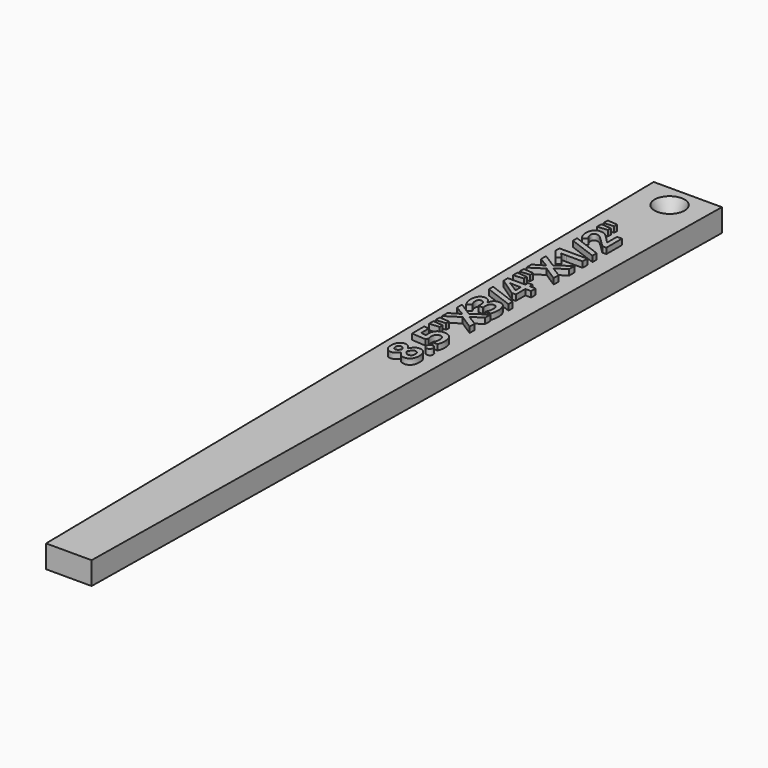
from build123d import *

# Parameters (mm, degrees)
F0_R         = 1.651
F1_DEPTH     = 6.35
F0_TEXT_SIZE = 10.8787272539
F2_DEPTH     = 1.5875
F3_SIZE2     = 2.54
F3_SIZE      = 5.842
F4_DEPTH     = 6.35


# Not quite as in the source:
# - Text() gives the source's letters only with a copy of the font that has no kerning and outlines rounded to 1/6400 em; it was checked with that copy


with BuildPart() as f1:
    # F0 (on Top) → F1 (new body)
    with BuildSketch(Plane.XY):
        Polygon((-35.2317076462, 101.3994294825), (-44.7541336775, 101.3994294825), (-54.2765597088, 101.3994294825), (-51.1044226587, -114.5005705175), (-44.7541336775, -114.5005705175), (-38.4038446963, -114.5005705175), align=None)
        Polygon((-48.8141954362, 16.2280014208), (-48.8141954362, 17.7102280092), (-46.0095235661, 17.490953663), (-46.0095235661, 16.4455759659), align=None, mode=Mode.SUBTRACT)
        Polygon((-48.8141954362, 18.4683393147), (-48.8141954362, 19.950565903), (-46.0095235661, 19.732991358), (-46.0095235661, 18.6876136609), align=None, mode=Mode.SUBTRACT)
        with BuildLine():
            add(Edge.make_bspline(
                [(-48.3994439597, 1.312246475), (-48.9144837031, 2.0023657352), (-48.9144837031, 3.1123358753)],
                knots=[0, 0, 0, 1, 1, 1], degree=2))
            add(Edge.make_bspline(
                [(-48.9144837031, 3.1123358753), (-48.9144837031, 4.22910522), (-48.4070930648, 4.911575375)],
                knots=[0, 0, 0, 1, 1, 1], degree=2))
            add(Edge.make_bspline(
                [(-48.4070930648, 4.911575375), (-47.8997024264, 5.5940455301), (-47.0396030529, 5.5940455301)],
                knots=[0, 0, 0, 1, 1, 1], degree=2))
            add(Edge.make_bspline(
                [(-47.0396030529, 5.5940455301), (-46.4446726562, 5.5940455301), (-45.9797770462, 5.2642841102)],
                knots=[0, 0, 0, 1, 1, 1], degree=2))
            add(Edge.make_bspline(
                [(-45.9797770462, 5.2642841102), (-45.5148814362, 4.9345226903), (-45.1494241926, 4.2019084018)],
                knots=[0, 0, 0, 1, 1, 1], degree=2))
            add(Edge.make_bspline(
                [(-45.1494241926, 4.2019084018), (-44.6819788809, 5.0722065821), (-44.1745882425, 5.4521121355)],
                knots=[0, 0, 0, 1, 1, 1], degree=2))
            add(Edge.make_bspline(
                [(-44.1745882425, 5.4521121355), (-43.6671976042, 5.8320176888), (-43.0603685996, 5.8320176888)],
                knots=[0, 0, 0, 1, 1, 1], degree=2))
            add(Edge.make_bspline(
                [(-43.0603685996, 5.8320176888), (-42.1050803626, 5.8320176888), (-41.5228984744, 5.0832552895)],
                knots=[0, 0, 0, 1, 1, 1], degree=2))
            add(Edge.make_bspline(
                [(-41.5228984744, 5.0832552895), (-40.9407165862, 4.3344928902), (-40.9407165862, 3.1123358753)],
                knots=[0, 0, 0, 1, 1, 1], degree=2))
            add(Edge.make_bspline(
                [(-40.9407165862, 3.1123358753), (-40.9407165862, 1.8374850252), (-41.4829531478, 1.1099701401)],
                knots=[0, 0, 0, 1, 1, 1], degree=2))
            add(Edge.make_bspline(
                [(-41.4829531478, 1.1099701401), (-42.0251897093, 0.382455255), (-43.0178735712, 0.382455255)],
                knots=[0, 0, 0, 1, 1, 1], degree=2))
            add(Edge.make_bspline(
                [(-43.0178735712, 0.382455255), (-43.6824958144, 0.382455255), (-44.1975355578, 0.7360138908)],
                knots=[0, 0, 0, 1, 1, 1], degree=2))
            add(Edge.make_bspline(
                [(-44.1975355578, 0.7360138908), (-44.7125753013, 1.0895725265), (-45.1069291642, 1.8697812468)],
                knots=[0, 0, 0, 1, 1, 1], degree=2))
            add(Edge.make_bspline(
                [(-45.1069291642, 1.8697812468), (-45.525080243, 1.2051590036), (-46.0035742621, 0.9136431092)],
                knots=[0, 0, 0, 1, 1, 1], degree=2))
            add(Edge.make_bspline(
                [(-46.0035742621, 0.9136431092), (-46.4820682812, 0.6221272148), (-47.0498018597, 0.6221272148)],
                knots=[0, 0, 0, 1, 1, 1], degree=2))
            add(Edge.make_bspline(
                [(-47.0498018597, 0.6221272148), (-47.8844042162, 0.6221272148), (-48.3994439597, 1.312246475)],
                knots=[0, 0, 0, 1, 1, 1], degree=2))
        make_face(mode=Mode.SUBTRACT)
        with BuildLine():
            add(Edge.make_bspline(
                [(-45.9347323162, 11.771122849), (-46.0095235661, 12.0957848655), (-46.0095235661, 12.573428984)],
                knots=[0, 0, 0, 1, 1, 1], degree=2))
            add(Edge.make_bspline(
                [(-46.0095235661, 12.573428984), (-46.0095235661, 13.6986973343), (-45.3771975444, 14.3658692792)],
                knots=[0, 0, 0, 1, 1, 1], degree=2))
            add(Edge.make_bspline(
                [(-45.3771975444, 14.3658692792), (-44.7448715228, 15.033041224), (-43.6451001895, 15.033041224)],
                knots=[0, 0, 0, 1, 1, 1], degree=2))
            add(Edge.make_bspline(
                [(-43.6451001895, 15.033041224), (-42.3447523224, 15.033041224), (-41.6427344543, 14.2307350891)],
                knots=[0, 0, 0, 1, 1, 1], degree=2))
            add(Edge.make_bspline(
                [(-41.6427344543, 14.2307350891), (-40.9407165862, 13.4284289541), (-40.9407165862, 11.9360035589)],
                knots=[0, 0, 0, 1, 1, 1], degree=2))
            add(Edge.make_bspline(
                [(-40.9407165862, 11.9360035589), (-40.9407165862, 10.6390552941), (-41.3605674661, 9.8435483637)],
                knots=[0, 0, 0, 1, 1, 1], degree=2))
            Line((-41.3605674661, 9.8435483637), (-42.7799014126, 9.8435483637))
            add(Edge.make_bspline(
                [(-42.7799014126, 9.8435483637), (-42.5572274641, 10.2616994425), (-42.41614397, 10.8200841148)],
                knots=[0, 0, 0, 1, 1, 1], degree=2))
            add(Edge.make_bspline(
                [(-42.41614397, 10.8200841148), (-42.2750604759, 11.3784687872), (-42.2750604759, 11.8765105193)],
                knots=[0, 0, 0, 1, 1, 1], degree=2))
            add(Edge.make_bspline(
                [(-42.2750604759, 11.8765105193), (-42.2750604759, 13.3808345223), (-43.5074162977, 13.3808345223)],
                knots=[0, 0, 0, 1, 1, 1], degree=2))
            add(Edge.make_bspline(
                [(-43.5074162977, 13.3808345223), (-44.6819788809, 13.3808345223), (-44.6819788809, 11.8238166841)],
                knots=[0, 0, 0, 1, 1, 1], degree=2))
            add(Edge.make_bspline(
                [(-44.6819788809, 11.8238166841), (-44.6819788809, 11.5433494971), (-44.6258854435, 11.2033892704)],
                knots=[0, 0, 0, 1, 1, 1], degree=2))
            add(Edge.make_bspline(
                [(-44.6258854435, 11.2033892704), (-44.5697920061, 10.8634290437), (-44.505199563, 10.6509539021)],
                knots=[0, 0, 0, 1, 1, 1], degree=2))
            Line((-44.505199563, 10.6509539021), (-44.8570583976, 9.9965304657))
            Line((-44.8570583976, 9.9965304657), (-48.8141954362, 10.2888962606))
            Line((-48.8141954362, 10.2888962606), (-48.8141954362, 14.5010034693))
            Line((-48.8141954362, 14.5010034693), (-47.422058308, 14.5010034693))
            Line((-47.422058308, 14.5010034693), (-47.422058308, 11.7286278207))
            Line((-47.422058308, 11.7286278207), (-45.8973366913, 11.5858445254))
            Line((-45.8973366913, 11.5858445254), (-45.9347323162, 11.771122849))
        make_face(mode=Mode.SUBTRACT)
        Polygon((-48.8141954362, 45.5342727623), (-48.8141954362, 47.0164993506), (-46.0095235661, 46.7972250044), (-46.0095235661, 45.7518473074), align=None, mode=Mode.SUBTRACT)
        Polygon((-44.9624460679, 25.2896412631), (-41.0478040576, 27.9141342132), (-41.0478040576, 26.0341541596), (-43.9850604162, 24.2272655548), (-41.0478040576, 22.4220767511), (-41.0478040576, 20.6576831746), (-45.052535528, 23.2345816928), (-48.8141954362, 20.8225638845), (-48.8141954362, 22.6396512961), (-46.0197223729, 24.3122556114), (-48.8141954362, 25.9542635063), (-48.8141954362, 27.7271560885), align=None, mode=Mode.SUBTRACT)
        with BuildLine():
            add(Edge.make_bspline(
                [(-48.435989684, 32.7772652559), (-47.9472968582, 33.4758835217), (-47.0769986779, 33.4758835217)],
                knots=[0, 0, 0, 1, 1, 1], degree=2))
            add(Edge.make_bspline(
                [(-47.0769986779, 33.4758835217), (-46.3494837928, 33.4758835217), (-45.8395434527, 33.0347851276)],
                knots=[0, 0, 0, 1, 1, 1], degree=2))
            add(Edge.make_bspline(
                [(-45.8395434527, 33.0347851276), (-45.3296031127, 32.5936867335), (-45.1375255846, 31.7964800019)],
                knots=[0, 0, 0, 1, 1, 1], degree=2))
            Line((-45.1375255846, 31.7964800019), (-45.1069291642, 31.7964800019))
            add(Edge.make_bspline(
                [(-45.1069291642, 31.7964800019), (-44.989642886, 32.7381698298), (-44.5349460828, 33.2209133517)],
                knots=[0, 0, 0, 1, 1, 1], degree=2))
            add(Edge.make_bspline(
                [(-44.5349460828, 33.2209133517), (-44.0802492796, 33.7036568736), (-43.3102393662, 33.7036568736)],
                knots=[0, 0, 0, 1, 1, 1], degree=2))
            add(Edge.make_bspline(
                [(-43.3102393662, 33.7036568736), (-42.1900704193, 33.7036568736), (-41.5653935027, 32.8911519318)],
                knots=[0, 0, 0, 1, 1, 1], degree=2))
            add(Edge.make_bspline(
                [(-41.5653935027, 32.8911519318), (-40.9407165862, 32.0786469901), (-40.9407165862, 30.5709233847)],
                knots=[0, 0, 0, 1, 1, 1], degree=2))
            add(Edge.make_bspline(
                [(-40.9407165862, 30.5709233847), (-40.9407165862, 29.3062713414), (-41.3605674661, 28.3288856897)],
                knots=[0, 0, 0, 1, 1, 1], degree=2))
            Line((-41.3605674661, 28.3288856897), (-42.7578039978, 28.3288856897))
            add(Edge.make_bspline(
                [(-42.7578039978, 28.3288856897), (-42.5300306459, 28.7793329901), (-42.3863974502, 29.3215695516)],
                knots=[0, 0, 0, 1, 1, 1], degree=2))
            add(Edge.make_bspline(
                [(-42.3863974502, 29.3215695516), (-42.2427642544, 29.8638061132), (-42.2427642544, 30.3941440668)],
                knots=[0, 0, 0, 1, 1, 1], degree=2))
            add(Edge.make_bspline(
                [(-42.2427642544, 30.3941440668), (-42.2427642544, 31.2083488097), (-42.5189819386, 31.5959034682)],
                knots=[0, 0, 0, 1, 1, 1], degree=2))
            add(Edge.make_bspline(
                [(-42.5189819386, 31.5959034682), (-42.7951996228, 31.9834581266), (-43.4071280308, 31.9834581266)],
                knots=[0, 0, 0, 1, 1, 1], degree=2))
            add(Edge.make_bspline(
                [(-43.4071280308, 31.9834581266), (-43.9527641946, 31.9834581266), (-44.1813874471, 31.5372603291)],
                knots=[0, 0, 0, 1, 1, 1], degree=2))
            add(Edge.make_bspline(
                [(-44.1813874471, 31.5372603291), (-44.4100106995, 31.0910625315), (-44.4100106995, 30.1136768798)],
                knots=[0, 0, 0, 1, 1, 1], degree=2))
            Line((-44.4100106995, 30.1136768798), (-44.4100106995, 29.5238458865))
            Line((-44.4100106995, 29.5238458865), (-45.6695633394, 29.5238458865))
            Line((-45.6695633394, 29.5238458865), (-45.6695633394, 30.1238756866))
            add(Edge.make_bspline(
                [(-45.6695633394, 30.1238756866), (-45.6695633394, 31.0264700885), (-45.9058356969, 31.4437712667)],
                knots=[0, 0, 0, 1, 1, 1], degree=2))
            add(Edge.make_bspline(
                [(-45.9058356969, 31.4437712667), (-46.1421080545, 31.861072445), (-46.7149410364, 31.861072445)],
                knots=[0, 0, 0, 1, 1, 1], degree=2))
            add(Edge.make_bspline(
                [(-46.7149410364, 31.861072445), (-47.5971378247, 31.861072445), (-47.5971378247, 30.7562017082)],
                knots=[0, 0, 0, 1, 1, 1], degree=2))
            add(Edge.make_bspline(
                [(-47.5971378247, 30.7562017082), (-47.5971378247, 30.3737464532), (-47.4696527397, 29.9776927891)],
                knots=[0, 0, 0, 1, 1, 1], degree=2))
            add(Edge.make_bspline(
                [(-47.4696527397, 29.9776927891), (-47.3421676547, 29.5816391251), (-47.0294042461, 29.0988956032)],
                knots=[0, 0, 0, 1, 1, 1], degree=2))
            Line((-47.0294042461, 29.0988956032), (-48.1597719999, 28.3390844965))
            add(Edge.make_bspline(
                [(-48.1597719999, 28.3390844965), (-48.9246825099, 29.4014602049), (-48.9246825099, 30.8734879865)],
                knots=[0, 0, 0, 1, 1, 1], degree=2))
            add(Edge.make_bspline(
                [(-48.9246825099, 30.8734879865), (-48.9246825099, 32.0786469901), (-48.435989684, 32.7772652559)],
                knots=[0, 0, 0, 1, 1, 1], degree=2))
        make_face(mode=Mode.SUBTRACT)
        Polygon((-48.8141954362, 37.0930603337), (-48.8141954362, 38.5650881152), (-41.0478040576, 35.6686269839), (-41.0478040576, 34.1982990034), align=None, mode=Mode.SUBTRACT)
        Polygon((-43.932366581, 44.6571753774), (-42.657515731, 44.6571753774), (-42.657515731, 43.722284754), (-41.0478040576, 43.722284754), (-41.0478040576, 42.1176724841), (-42.657515731, 42.1176724841), (-42.657515731, 38.8030602739), (-43.7997820926, 38.8030602739), (-48.8141954362, 42.2094617453), (-48.8141954362, 43.722284754), (-43.932366581, 43.722284754), align=None, mode=Mode.SUBTRACT)
        Polygon((-48.8141954362, 47.7746106561), (-48.8141954362, 49.2568372445), (-46.0095235661, 49.0392626994), (-46.0095235661, 47.9938850023), align=None, mode=Mode.SUBTRACT)
        Polygon((-44.9624460679, 54.5959126046), (-41.0478040576, 57.2204055546), (-41.0478040576, 55.340425501), (-43.9850604162, 53.5335368962), (-41.0478040576, 51.7283480925), (-41.0478040576, 49.963954516), (-45.052535528, 52.5408530343), (-48.8141954362, 50.1288352259), (-48.8141954362, 51.9459226376), (-46.0197223729, 53.6185269529), (-48.8141954362, 55.2605348478), (-48.8141954362, 57.0334274299), align=None, mode=Mode.SUBTRACT)
        with BuildLine():
            Line((-48.8141954362, 61.7146797514), (-41.0478040576, 61.7146797514))
            Line((-41.0478040576, 61.7146797514), (-41.0478040576, 60.0726718565))
            Line((-41.0478040576, 60.0726718565), (-45.5420782544, 60.0726718565))
            Line((-45.5420782544, 60.0726718565), (-46.2797919463, 60.0896698678))
            Line((-46.2797919463, 60.0896698678), (-47.0871974847, 60.1151668848))
            add(Edge.make_bspline(
                [(-47.0871974847, 60.1151668848), (-46.6792452126, 59.7072146128), (-46.5517601276, 59.5474333063)],
                knots=[0, 0, 0, 1, 1, 1], degree=2))
            Line((-46.5517601276, 59.5474333063), (-45.8344440493, 58.6550377112))
            Line((-45.8344440493, 58.6550377112), (-46.8220285079, 57.862930383))
            Line((-46.8220285079, 57.862930383), (-48.8141954362, 60.3650376514))
            Line((-48.8141954362, 60.3650376514), (-48.8141954362, 61.7146797514))
        make_face(mode=Mode.SUBTRACT)
        Polygon((-48.8141954362, 66.3993316751), (-48.8141954362, 67.8713594567), (-41.0478040576, 64.9748983253), (-41.0478040576, 63.5045703449), align=None, mode=Mode.SUBTRACT)
        with BuildLine():
            Line((-42.4297423791, 73.7883672021), (-41.0478040576, 73.7883672021))
            Line((-41.0478040576, 73.7883672021), (-41.0478040576, 68.3592023819))
            Line((-41.0478040576, 68.3592023819), (-42.1900704193, 68.3592023819))
            Line((-42.1900704193, 68.3592023819), (-44.1601399329, 70.308874282))
            add(Edge.make_bspline(
                [(-44.1601399329, 70.308874282), (-45.0474361246, 71.17577286), (-45.3899460529, 71.4409418369)],
                knots=[0, 0, 0, 1, 1, 1], degree=2))
            add(Edge.make_bspline(
                [(-45.3899460529, 71.4409418369), (-45.7324559813, 71.7061108137), (-46.0248217763, 71.8233970919)],
                knots=[0, 0, 0, 1, 1, 1], degree=2))
            add(Edge.make_bspline(
                [(-46.0248217763, 71.8233970919), (-46.3171875712, 71.9406833701), (-46.6299509798, 71.9406833701)],
                knots=[0, 0, 0, 1, 1, 1], degree=2))
            add(Edge.make_bspline(
                [(-46.6299509798, 71.9406833701), (-47.0973962915, 71.9406833701), (-47.3260195439, 71.6823135978)],
                knots=[0, 0, 0, 1, 1, 1], degree=2))
            add(Edge.make_bspline(
                [(-47.3260195439, 71.6823135978), (-47.5546427964, 71.4239438255), (-47.5546427964, 70.9938941388)],
                knots=[0, 0, 0, 1, 1, 1], degree=2))
            add(Edge.make_bspline(
                [(-47.5546427964, 70.9938941388), (-47.5546427964, 70.5434468384), (-47.3472670581, 70.118496555)],
                knots=[0, 0, 0, 1, 1, 1], degree=2))
            add(Edge.make_bspline(
                [(-47.3472670581, 70.118496555), (-47.1398913198, 69.6935462717), (-46.7574360648, 69.2312003634)],
                knots=[0, 0, 0, 1, 1, 1], degree=2))
            Line((-46.7574360648, 69.2312003634), (-47.8147123698, 68.3388047683))
            add(Edge.make_bspline(
                [(-47.8147123698, 68.3388047683), (-48.3042550962, 68.9116377503), (-48.5056815305, 69.2889936019)],
                knots=[0, 0, 0, 1, 1, 1], degree=2))
            add(Edge.make_bspline(
                [(-48.5056815305, 69.2889936019), (-48.7071079648, 69.6663494536), (-48.8158952374, 70.1125472511)],
                knots=[0, 0, 0, 1, 1, 1], degree=2))
            add(Edge.make_bspline(
                [(-48.8158952374, 70.1125472511), (-48.9246825099, 70.5587450486), (-48.9246825099, 71.111180417)],
                knots=[0, 0, 0, 1, 1, 1], degree=2))
            add(Edge.make_bspline(
                [(-48.9246825099, 71.111180417), (-48.9246825099, 71.8386953021), (-48.6595135331, 72.3962300738)],
                knots=[0, 0, 0, 1, 1, 1], degree=2))
            add(Edge.make_bspline(
                [(-48.6595135331, 72.3962300738), (-48.3943445563, 72.9537648456), (-47.9158505372, 73.2622787513)],
                knots=[0, 0, 0, 1, 1, 1], degree=2))
            add(Edge.make_bspline(
                [(-47.9158505372, 73.2622787513), (-47.4373565182, 73.570792657), (-46.8220285079, 73.570792657)],
                knots=[0, 0, 0, 1, 1, 1], degree=2))
            add(Edge.make_bspline(
                [(-46.8220285079, 73.570792657), (-46.2848913497, 73.570792657), (-45.8148963363, 73.3821147312)],
                knots=[0, 0, 0, 1, 1, 1], degree=2))
            add(Edge.make_bspline(
                [(-45.8148963363, 73.3821147312), (-45.3449013229, 73.1934368054), (-44.8511090936, 72.7973831413)],
                knots=[0, 0, 0, 1, 1, 1], degree=2))
            add(Edge.make_bspline(
                [(-44.8511090936, 72.7973831413), (-44.3573168644, 72.4013294772), (-43.4428238546, 71.4035462119)],
                knots=[0, 0, 0, 1, 1, 1], degree=2))
            Line((-43.4428238546, 71.4035462119), (-42.5028338278, 70.4040631455))
            Line((-42.5028338278, 70.4040631455), (-42.4297423791, 70.4040631455))
            Line((-42.4297423791, 70.4040631455), (-42.4297423791, 73.7883672021))
        make_face(mode=Mode.SUBTRACT)
        Polygon((-48.8141954362, 74.8405441037), (-48.8141954362, 76.3227706921), (-46.0095235661, 76.1034963458), (-46.0095235661, 75.0581186488), align=None, mode=Mode.SUBTRACT)
        Polygon((-48.8141954362, 77.0808819976), (-48.8141954362, 78.5631085859), (-46.0095235661, 78.3455340408), (-46.0095235661, 77.3001563438), align=None, mode=Mode.SUBTRACT)
        with BuildLine():
            add(Edge.make_bspline(
                [(-41.1412931199, 7.0754222179), (-41.3775654775, 6.8315007552), (-41.8076151642, 6.8315007552)],
                knots=[0, 0, 0, 1, 1, 1], degree=2))
            add(Edge.make_bspline(
                [(-41.8076151642, 6.8315007552), (-42.2529630612, 6.8315007552), (-42.4815863136, 7.0703228145)],
                knots=[0, 0, 0, 1, 1, 1], degree=2))
            add(Edge.make_bspline(
                [(-42.4815863136, 7.0703228145), (-42.7102095661, 7.3091448737), (-42.7102095661, 7.7663913786)],
                knots=[0, 0, 0, 1, 1, 1], degree=2))
            add(Edge.make_bspline(
                [(-42.7102095661, 7.7663913786), (-42.7102095661, 8.2066398722), (-42.4764869102, 8.4480116331)],
                knots=[0, 0, 0, 1, 1, 1], degree=2))
            add(Edge.make_bspline(
                [(-42.4764869102, 8.4480116331), (-42.2427642544, 8.6893833941), (-41.8076151642, 8.6893833941)],
                knots=[0, 0, 0, 1, 1, 1], degree=2))
            add(Edge.make_bspline(
                [(-41.8076151642, 8.6893833941), (-41.3877642843, 8.6893833941), (-41.1463925233, 8.4454619314)],
                knots=[0, 0, 0, 1, 1, 1], degree=2))
            add(Edge.make_bspline(
                [(-41.1463925233, 8.4454619314), (-40.9050207624, 8.2015404688), (-40.9050207624, 7.7663913786)],
                knots=[0, 0, 0, 1, 1, 1], degree=2))
            add(Edge.make_bspline(
                [(-40.9050207624, 7.7663913786), (-40.9050207624, 7.3193436805), (-41.1412931199, 7.0754222179)],
                knots=[0, 0, 0, 1, 1, 1], degree=2))
        make_face(mode=Mode.SUBTRACT)
        with Locations((-44.7541336775, 95.0494294825)):
            Circle(F0_R, mode=Mode.SUBTRACT)
    extrude(amount=-F1_DEPTH)

    # F3
    f3_edges = [f1.edges().sort_by_distance(p)[0] for p in [
        (-46.405134, 95.049429, 0),
    ]]
    f3_side = f1.faces().sort_by_distance((-46.405134, 95.049429, -3.175))[0]
    chamfer(f3_edges, length=F3_SIZE, length2=F3_SIZE2, reference=f3_side)


with BuildPart() as f2:
    # F0 (on Top) → F2 (new body)
    with BuildSketch(Plane.XY):
        with Locations(Location((-41.0478040576, 0), (0, 0, 90))):
            Text('8.5"X3/4"X1/2"', F0_TEXT_SIZE, font='Open Sans', font_style=FontStyle.BOLD, text_align=(TextAlign.LEFT, TextAlign.BOTTOM))
    extrude(amount=F2_DEPTH)


with BuildPart() as f4:
    # F0 (on Top) → F4 (new body)
    with BuildSketch(Plane.XY):
        with BuildLine():
            add(Edge.make_bspline(
                [(-44.4321081143, 3.032445222), (-43.9102691663, 1.9020774683), (-43.1147622358, 1.9020774683)],
                knots=[0, 0, 0, 1, 1, 1], degree=2))
            add(Edge.make_bspline(
                [(-43.1147622358, 1.9020774683), (-42.657515731, 1.9020774683), (-42.4025455609, 2.2207901808)],
                knots=[0, 0, 0, 1, 1, 1], degree=2))
            add(Edge.make_bspline(
                [(-42.4025455609, 2.2207901808), (-42.1475753909, 2.5395028933), (-42.1475753909, 3.0919382617)],
                knots=[0, 0, 0, 1, 1, 1], degree=2))
            add(Edge.make_bspline(
                [(-42.1475753909, 3.0919382617), (-42.1475753909, 3.7021668686), (-42.410194666, 4.0047314704)],
                knots=[0, 0, 0, 1, 1, 1], degree=2))
            add(Edge.make_bspline(
                [(-42.410194666, 4.0047314704), (-42.6728139412, 4.3072960721), (-43.1028636279, 4.3072960721)],
                knots=[0, 0, 0, 1, 1, 1], degree=2))
            add(Edge.make_bspline(
                [(-43.1028636279, 4.3072960721), (-43.4598218659, 4.3072960721), (-43.7700355728, 4.0072811721)],
                knots=[0, 0, 0, 1, 1, 1], degree=2))
            add(Edge.make_bspline(
                [(-43.7700355728, 4.0072811721), (-44.0802492796, 3.707266272), (-44.4321081143, 3.032445222)],
                knots=[0, 0, 0, 1, 1, 1], degree=2))
        make_face()
        with Locations(Location((-41.0478040576, 0), (0, 0, 90))):
            Text('8.5"X3/4"X1/2"', F0_TEXT_SIZE, font='Open Sans', font_style=FontStyle.BOLD, text_align=(TextAlign.LEFT, TextAlign.BOTTOM))
        with BuildLine():
            Line((-43.932366581, 40.2478912373), (-43.932366581, 42.1176724841))
            Line((-43.932366581, 42.1176724841), (-45.2497124594, 42.1176724841))
            add(Edge.make_bspline(
                [(-45.2497124594, 42.1176724841), (-45.5794738793, 42.1176724841), (-46.205850597, 42.1448693022)],
                knots=[0, 0, 0, 1, 1, 1], degree=2))
            add(Edge.make_bspline(
                [(-46.205850597, 42.1448693022), (-46.8322273147, 42.1720661204), (-46.9342153827, 42.1873643306)],
                knots=[0, 0, 0, 1, 1, 1], degree=2))
            Line((-46.9342153827, 42.1873643306), (-46.9342153827, 42.1448693022))
            add(Edge.make_bspline(
                [(-46.9342153827, 42.1448693022), (-46.4973664914, 41.9476923707), (-46.0843148159, 41.6723245871)],
                knots=[0, 0, 0, 1, 1, 1], degree=2))
            Line((-46.0843148159, 41.6723245871), (-43.932366581, 40.2478912373))
        make_face()
        with BuildLine():
            add(Edge.make_bspline(
                [(-47.5019489612, 3.7820575219), (-47.7144241029, 3.5168885451), (-47.7144241029, 3.1021370685)],
                knots=[0, 0, 0, 1, 1, 1], degree=2))
            add(Edge.make_bspline(
                [(-47.7144241029, 3.1021370685), (-47.7144241029, 2.6822861885), (-47.4993992595, 2.4247663168)],
                knots=[0, 0, 0, 1, 1, 1], degree=2))
            add(Edge.make_bspline(
                [(-47.4993992595, 2.4247663168), (-47.2843744161, 2.1672464451), (-46.9223167747, 2.1672464451)],
                knots=[0, 0, 0, 1, 1, 1], degree=2))
            add(Edge.make_bspline(
                [(-46.9223167747, 2.1672464451), (-46.6044539628, 2.1672464451), (-46.3520334945, 2.3720724817)],
                knots=[0, 0, 0, 1, 1, 1], degree=2))
            add(Edge.make_bspline(
                [(-46.3520334945, 2.3720724817), (-46.0996130261, 2.5768985183), (-45.8344440493, 3.1123358753)],
                knots=[0, 0, 0, 1, 1, 1], degree=2))
            add(Edge.make_bspline(
                [(-45.8344440493, 3.1123358753), (-46.0775156114, 3.6341748233), (-46.3324857814, 3.840700661)],
                knots=[0, 0, 0, 1, 1, 1], degree=2))
            add(Edge.make_bspline(
                [(-46.3324857814, 3.840700661), (-46.5874559514, 4.0472264987), (-46.9223167747, 4.0472264987)],
                knots=[0, 0, 0, 1, 1, 1], degree=2))
            add(Edge.make_bspline(
                [(-46.9223167747, 4.0472264987), (-47.2894738195, 4.0472264987), (-47.5019489612, 3.7820575219)],
                knots=[0, 0, 0, 1, 1, 1], degree=2))
        make_face()
    extrude(amount=-F4_DEPTH)


solid = Compound([f1.part, f2.part, f4.part])
